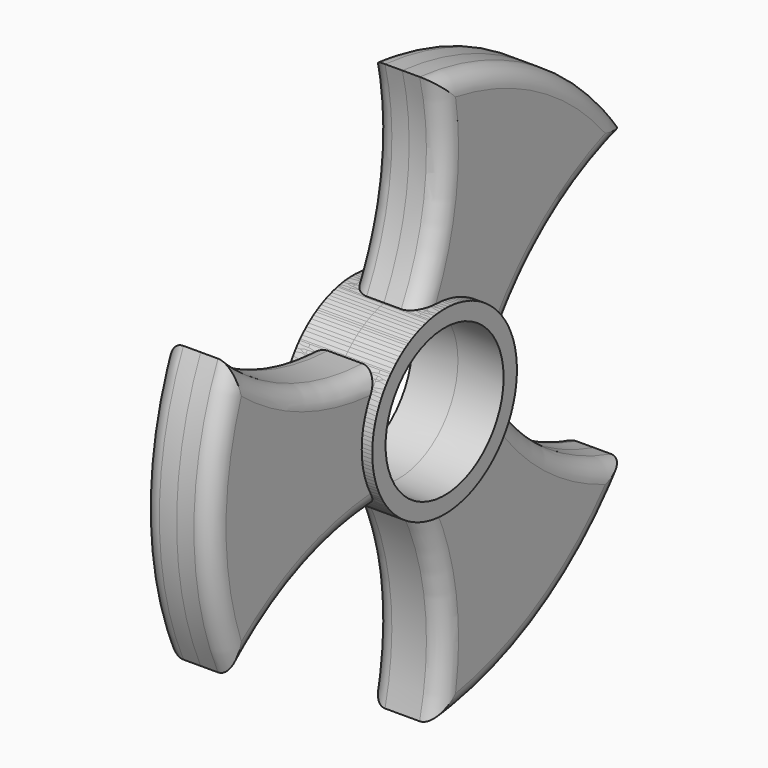
from build123d import *

# Parameters (mm, degrees)
F0_R          = 10.5
F1_DEPTH      = 6.5
F1_DEPTH_BACK = 6.5
F2_DEPTH      = 5
F2_DEPTH_BACK = 5
F3_T4_ANGLE   = 60.6424009428
F3_S5_R       = 12.8699040868
F3_T6_DEPTH   = 26
F3_T10_ANGLE  = 60.6424009428
F3_S11_R      = 12.8699040868
F3_T12_DEPTH  = 25
F3_T14_ANGLE  = 64.5478705819
F3_T18_ANGLE  = 60.6424009428
F3_S19_R      = 12.8699040868
F3_T20_DEPTH  = 26
F3_T22_ANGLE  = 64.5478705819
F3_T26_ANGLE  = 60.6424009428
F3_S27_R      = 12.8699040868
F3_T28_DEPTH  = 26
F4_COUNT      = 3


# Not quite as in the source:
# - a fillet or chamfer that OpenCascade refuses, or shapes differently, is made with other operations: its cross-section is extruded or revolved along the edge and cut away or added


with BuildPart() as f1:
    # F0 (on Right) → F1 (new body, two sides)
    with BuildSketch(Plane.YZ) as f1_sk:
        with BuildLine():
            ThreePointArc((-9.5784175244, -8.5958332307), (4.6022340423, -12.0188964977), (12.8699040868, 0))
            ThreePointArc((12.8699040868, 0), (4.6022340423, 12.0188964977), (-9.5784175244, 8.5958332307))
            ThreePointArc((-9.5784175244, 8.5958332307), (-12.8699040868, 0), (-9.5784175244, -8.5958332307))
        make_face()
        Circle(F0_R, mode=Mode.SUBTRACT)
    extrude(amount=F1_DEPTH)
    extrude(f1_sk.sketch, amount=-F1_DEPTH_BACK)

    # F0 (on Right) → F2 (join, two sides)
    with BuildSketch(Plane.YZ) as f2_sk:
        with BuildLine():
            ThreePointArc((-9.5784175244, -8.5958332307), (-12.8699040868, 0), (-9.5784175244, 8.5958332307))
            ThreePointArc((-9.5784175244, 8.5958332307), (-23.4502453241, 11.7471070447), (-35.2715310157, 19.6600924328))
            ThreePointArc((-35.2715310157, 19.6600924328), (-39.5538669274, 0), (-35.2715310157, -19.6600924328))
            ThreePointArc((-35.2715310157, -19.6600924328), (-23.4502453241, -11.7471070447), (-9.5784175244, -8.5958332307))
        make_face()
    extrude(amount=F2_DEPTH)
    extrude(f2_sk.sketch, amount=-F2_DEPTH_BACK)

    # F3: fillet of radius 2.54 on 6 edges, made by hand


with BuildPart() as f3_tool2:
    # F3_s3 → F3_t4 (revolve)
    with BuildSketch(Plane(origin=(0, -2.1169859071, -0.2607949346), x_dir=(1, 0, 0), z_dir=(0, 0.9924972024, 0.1222673434))):
        with BuildLine():
            ThreePointArc((2.46, -9.1869808052), (4.2560512242, -8.4430320294), (5, -6.6469808052))
            Line((5, -6.6469808052), (5, -9.1869808052))
            Line((5, -9.1869808052), (2.46, -9.1869808052))
        make_face()
    revolve(axis=Axis((5, -8.0125527589, 47.5960852616), (-1, 0, 0)), revolution_arc=F3_T4_ANGLE)

    # F3_s5 → F3_t6 (cut, symmetric)
    with BuildSketch(Plane.YZ.offset(2.8)):
        Circle(F3_S5_R)
    extrude(amount=F3_T6_DEPTH, both=True, mode=Mode.SUBTRACT)


with BuildPart() as f1_1:
    add(f1.part)

    # F3_t1: cut F3_tool2
    add(f3_tool2.part, mode=Mode.SUBTRACT)


with BuildPart() as f3_tool8:
    # F3_s9 → F3_t10 (revolve)
    with BuildSketch(Plane(origin=(0, -25.5479715761, -34.6770339233), x_dir=(1, 0, 0), z_dir=(0, -0.5931459635, -0.8050949422))):
        with BuildLine():
            ThreePointArc((5, 19.7911140481), (4.2560512242, 17.9950628239), (2.46, 17.2511140481))
            Line((2.46, 17.2511140481), (5, 17.2511140481))
            Line((5, 17.2511140481), (5, 19.7911140481))
        make_face()
    revolve(axis=Axis((5, -8.0125527589, -47.5960852616), (-1, 0, 0)), revolution_arc=F3_T10_ANGLE)

    # F3_s11 → F3_t12 (cut, symmetric)
    with BuildSketch(Plane.YZ.offset(2.8)):
        Circle(F3_S11_R)
    extrude(amount=F3_T12_DEPTH, both=True, mode=Mode.SUBTRACT)


with BuildPart() as f1_2:
    add(f1_1.part)

    # F3_t7: cut F3_tool8
    add(f3_tool8.part, mode=Mode.SUBTRACT)

    # F3_s13 → F3_t14 (revolve, cut)
    with BuildSketch(Plane(origin=(0, 2.2002224312, 3.4839156822), x_dir=(1, 0, 0), z_dir=(0, 0.5339677718, 0.8455048306))):
        with BuildLine():
            ThreePointArc((2.46, -40.7460731978), (4.2560512242, -40.002124422), (5, -38.2060731978))
            Line((5, -38.2060731978), (5, -40.7460731978))
            Line((5, -40.7460731978), (2.46, -40.7460731978))
        make_face()
    revolve(axis=Axis((5, 7.7167867152, 0), (1, 0, 0)), revolution_arc=F3_T14_ANGLE, mode=Mode.SUBTRACT)


with BuildPart() as f3_tool16:
    # F3_s17 → F3_t18 (revolve)
    with BuildSketch(Plane(origin=(0, -2.1169859071, -0.2607949346), x_dir=(1, 0, 0), z_dir=(0, 0.9924972024, 0.1222673434))):
        with BuildLine():
            ThreePointArc((-2.46, -9.1869808052), (-4.2560512242, -8.4430320294), (-5, -6.6469808052))
            Line((-5, -6.6469808052), (-5, -9.1869808052))
            Line((-5, -9.1869808052), (-2.46, -9.1869808052))
        make_face()
    revolve(axis=Axis((-5, -8.0125527589, 47.5960852616), (-1, 0, 0)), revolution_arc=F3_T18_ANGLE)

    # F3_s19 → F3_t20 (cut, symmetric)
    with BuildSketch(Plane.YZ.offset(-2.8)):
        Circle(F3_S19_R)
    extrude(amount=F3_T20_DEPTH, both=True, mode=Mode.SUBTRACT)


with BuildPart() as f1_3:
    add(f1_2.part)

    # F3_t15: cut F3_tool16
    add(f3_tool16.part, mode=Mode.SUBTRACT)

    # F3_s21 → F3_t22 (revolve, cut)
    with BuildSketch(Plane(origin=(0, 2.2002224312, 3.4839156822), x_dir=(1, 0, 0), z_dir=(0, 0.5339677718, 0.8455048306))):
        with BuildLine():
            ThreePointArc((-2.46, -40.7460731978), (-4.2560512242, -40.002124422), (-5, -38.2060731978))
            Line((-5, -38.2060731978), (-5, -40.7460731978))
            Line((-5, -40.7460731978), (-2.46, -40.7460731978))
        make_face()
    revolve(axis=Axis((-5, 7.7167867152, 0), (1, 0, 0)), revolution_arc=F3_T22_ANGLE, mode=Mode.SUBTRACT)


with BuildPart() as f3_tool24:
    # F3_s25 → F3_t26 (revolve)
    with BuildSketch(Plane(origin=(0, -25.5479715761, -34.6770339233), x_dir=(1, 0, 0), z_dir=(0, -0.5931459635, -0.8050949422))):
        with BuildLine():
            ThreePointArc((-2.46, 17.2511140481), (-4.2560512242, 17.9950628239), (-5, 19.7911140481))
            Line((-5, 19.7911140481), (-5, 17.2511140481))
            Line((-5, 17.2511140481), (-2.46, 17.2511140481))
        make_face()
    revolve(axis=Axis((-5, -8.0125527589, -47.5960852616), (-1, 0, 0)), revolution_arc=F3_T26_ANGLE)

    # F3_s27 → F3_t28 (cut, symmetric)
    with BuildSketch(Plane.YZ.offset(-2.8)):
        Circle(F3_S27_R)
    extrude(amount=F3_T28_DEPTH, both=True, mode=Mode.SUBTRACT)


with BuildPart() as f1_4:
    add(f1_3.part)

    # F3_t23: cut F3_tool24
    add(f3_tool24.part, mode=Mode.SUBTRACT)


with BuildPart() as f4_1:
    # F4: instance of F1
    add(f1_4.part.rotate(Axis((6.5, 0, 0), (-1, 0, 0)), 1 * 360 / F4_COUNT))


with BuildPart() as f4_2:
    # F4: instance of F1
    add(f1_4.part.rotate(Axis((6.5, 0, 0), (-1, 0, 0)), 2 * 360 / F4_COUNT))


solid = Compound([f1_4.part, f4_1.part, f4_2.part])
